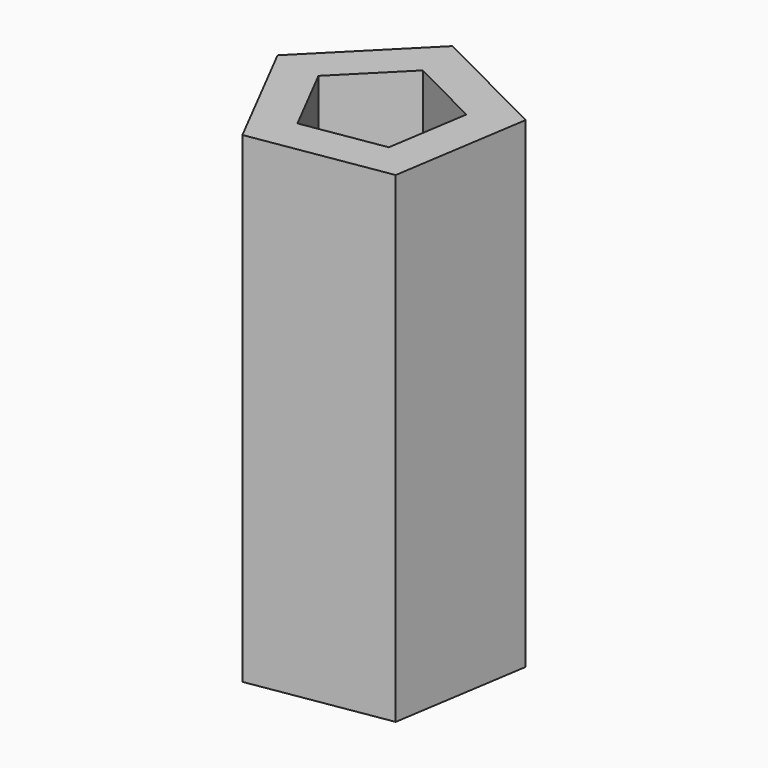
from build123d import *

# Parameters (mm, degrees)
F1_DEPTH = 177.8
F2_T     = -14.1111111111


# Not quite as in the source:
# - a length typed as a fraction of an inch, garbled in the dataset ("3 / 203.2 mm" for 3/8 in), is restored


with BuildPart() as f1:
    # F0 (on Top) → F1 (new body)
    with BuildSketch(Plane.XY):
        Polygon((-6.8708224943, 42.663338416), (-42.6984469235, 6.6491561018), (-19.5182689713, -38.5539339486), (30.6354932977, -30.4767976821), (38.4520450914, 19.7182371128), align=None)
    extrude(amount=F1_DEPTH)

    # F2
    f2_openings = [f1.faces().sort_by_distance(p)[0] for p in [
        (0, 0, 177.8),
    ]]
    offset(amount=F2_T, openings=f2_openings)


solid = f1.part
